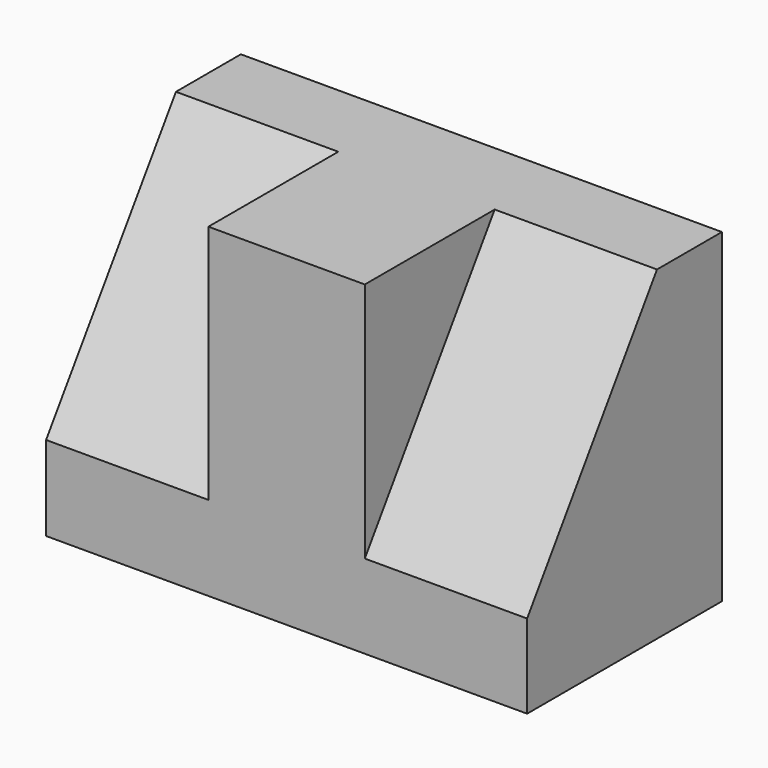
from build123d import *

# Parameters (mm, degrees)
F0_W     = 150.5499258637
F0_H     = 101.7426103354
F1_DEPTH = 50.8
F3_DEPTH = 50.8
F5_DEPTH = 50.8
F7_DEPTH = 25.4


with BuildPart() as f1:
    # F0 (on Front) → F1 (new body)
    with BuildSketch(Plane.XZ):
        with Locations((-0.8498765528, 5.2206814289)):
            Rectangle(F0_W, F0_H)
    extrude(amount=F1_DEPTH)

    # F2 (on face) → F3 (cut)
    with BuildSketch(Plane(origin=(-76.1248394847, 0, 0), x_dir=(0, -1, 0), z_dir=(-1, 0, 0))):
        Polygon((0, 56.0919865966), (50.8, -19.1829744726), (50.8, 56.0919865966), align=None)
    extrude(amount=-F3_DEPTH, mode=Mode.SUBTRACT)

    # F4 (on face) → F5 (cut)
    with BuildSketch(Plane.YZ.offset(74.4250863791)):
        Polygon((-50.8, 56.0919865966), (-50.8, -19.4257982075), (0, 56.0919865966), align=None)
    extrude(amount=-F5_DEPTH, mode=Mode.SUBTRACT)

    # F6 (on face) → F7 (join)
    with BuildSketch(Plane(origin=(0, 0, 0), x_dir=(-1, 0, 0), z_dir=(0, 1, 0))):
        Polygon((-23.6250863791, 56.0919865966), (-74.4250863791, 56.0919865966), (-74.4250863791, -45.6506237388), (76.1248394847, -45.6506237388), (76.1248394847, 56.0919865966), (25.3248394847, 56.0919865966), align=None)
    extrude(amount=F7_DEPTH)


solid = f1.part
